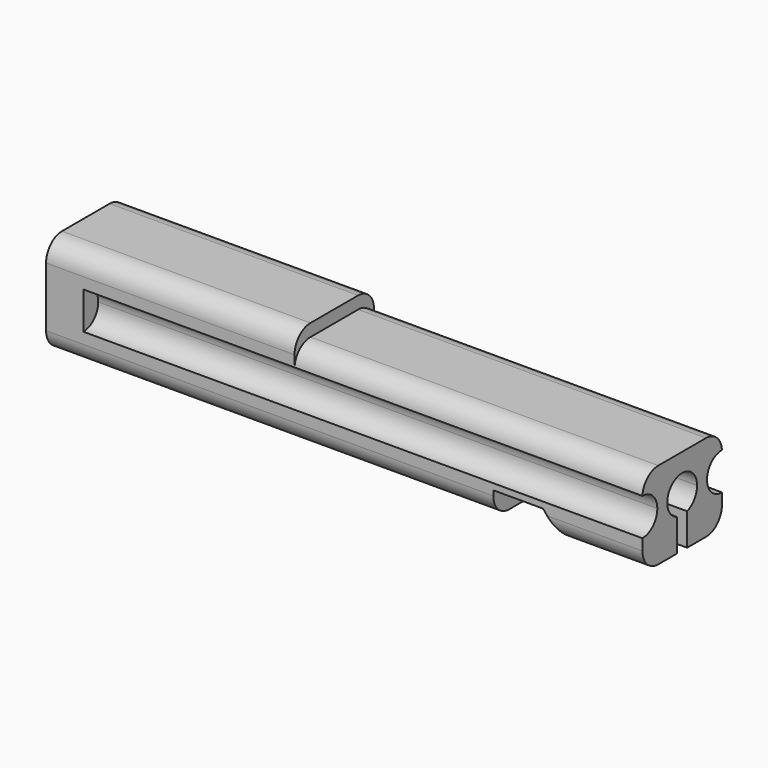
from build123d import *

# Parameters (mm, degrees)
F0_W        = 142.875
F0_H        = 9.525
F1_DEPTH    = 12.7
F3_DEPTH    = 142.875
F5_DEPTH    = 9.525
F6_DEPTH    = 142.875
F7_T1_DEPTH = 101.5751710417
F7_T3_DEPTH = 45.552419836
F7_T5_DEPTH = 139.7
F8_R        = 5.08
F9_DEPTH    = 60.325


# Not quite as in the source:
# - a fillet or chamfer that OpenCascade refuses, or shapes differently, is made with other operations: its cross-section is extruded or revolved along the edge and cut away or added


with BuildPart() as f1:
    # F0 (on Front) → F1 (new body, symmetric)
    with BuildSketch(Plane.XZ):
        Polygon((-20.4177256674, 25.4), (-83.9177256674, 25.4), (-83.9177256674, 0), (30.3822743326, 0), (30.3822743326, 6.35), (43.0822743326, 6.35), (48.3298544966, 0), (68.4822743326, 0), (68.4822743326, 7.9375), (-74.3927256674, 7.9375), (-74.3927256674, 17.4625), (68.4822743326, 17.4625), (68.4822743326, 22.225), (-20.4177256674, 22.225), align=None)
        with Locations((-2.9552256674, 12.7)):
            Rectangle(F0_W, F0_H)
    extrude(amount=F1_DEPTH, both=True)

    # F2 (on face) → F3 (cut)
    with BuildSketch(Plane.YZ.offset(68.4822743326)):
        with BuildLine():
            Line((-4.7625, 12.7), (0, 12.7))
            Line((0, 12.7), (4.7625, 12.7))
            ThreePointArc((4.7625, 12.7), (0, 17.4625), (-4.7625, 12.7))
        make_face()
        with BuildLine():
            Line((-1.5875, 8.2098719395), (0, 8.2098719395))
            Line((0, 8.2098719395), (0, 12.7))
            Line((0, 12.7), (-4.7625, 12.7))
            ThreePointArc((-4.7625, 12.7), (-3.8885649667, 9.950369343), (-1.5875, 8.2098719395))
        make_face()
        with BuildLine():
            ThreePointArc((-1.5875, 8.2098719395), (-0.8053481737, 8.0060868597), (0, 7.9375))
            Line((0, 7.9375), (0, 8.2098719395))
            Line((0, 8.2098719395), (-1.5875, 8.2098719395))
        make_face()
        with BuildLine():
            Line((0, 8.2098719395), (0, 7.9375))
            ThreePointArc((0, 7.9375), (0.8053481737, 8.0060868597), (1.5875, 8.2098719395))
            Line((1.5875, 8.2098719395), (0, 8.2098719395))
        make_face()
        with BuildLine():
            Line((0, 12.7), (0, 8.2098719395))
            Line((0, 8.2098719395), (1.5875, 8.2098719395))
            ThreePointArc((1.5875, 8.2098719395), (3.8885649667, 9.950369343), (4.7625, 12.7))
            Line((4.7625, 12.7), (0, 12.7))
        make_face()
    extrude(amount=-F3_DEPTH, mode=Mode.SUBTRACT)

    # F4 (on face) → F5 (cut)
    with BuildSketch(Plane(origin=(-83.9177256674, 0, 0), x_dir=(0, -1, 0), z_dir=(-1, 0, 0))):
        with BuildLine():
            Line((-0.79375, 12.7), (0.79375, 12.7))
            ThreePointArc((0.79375, 12.7), (0, 13.49375), (-0.79375, 12.7))
        make_face()
        with BuildLine():
            ThreePointArc((-0.79375, 12.7), (0, 11.90625), (0.79375, 12.7))
            Line((0.79375, 12.7), (-0.79375, 12.7))
        make_face()
    extrude(amount=-F5_DEPTH, mode=Mode.SUBTRACT)

    # F2 (on face) → F6 (cut)
    with BuildSketch(Plane.YZ.offset(68.4822743326)):
        with BuildLine():
            ThreePointArc((12.7, 17.4625), (9.3324039546, 16.0675960454), (7.9375, 12.7))
            Line((7.9375, 12.7), (12.7, 12.7))
            Line((12.7, 12.7), (12.7, 17.4625))
        make_face()
        with BuildLine():
            ThreePointArc((7.9375, 12.7), (9.3324039546, 9.3324039546), (12.7, 7.9375))
            Line((12.7, 7.9375), (12.7, 12.7))
            Line((12.7, 12.7), (7.9375, 12.7))
        make_face()
        with BuildLine():
            Line((-12.7, 12.7), (-12.7, 7.9375))
            ThreePointArc((-12.7, 7.9375), (-9.3324039546, 9.3324039546), (-7.9375, 12.7))
            Line((-7.9375, 12.7), (-12.7, 12.7))
        make_face()
        with BuildLine():
            Line((-12.7, 12.7), (-7.9375, 12.7))
            ThreePointArc((-7.9375, 12.7), (-9.3324039546, 16.0675960454), (-12.7, 17.4625))
            Line((-12.7, 17.4625), (-12.7, 12.7))
        make_face()
    extrude(amount=-F6_DEPTH, mode=Mode.SUBTRACT)

    # F7: fillet of radius 5.08 on 6 edges, made by hand

    # F7_s2 → F7_t1 (cut)
    with BuildSketch(Plane.YZ.offset(-20.4177256674)):
        with BuildLine():
            ThreePointArc((7.6299315833, 22.225), (11.1079698235, 20.8476544532), (12.7, 17.4625))
            Line((12.7, 17.4625), (12.7, 22.225))
            Line((12.7, 22.225), (7.6299315833, 22.225))
        make_face()
        with BuildLine():
            ThreePointArc((-7.6299315833, 22.225), (-11.1079698235, 20.8476544532), (-12.7, 17.4625))
            Line((-12.7, 17.4625), (-12.7, 22.225))
            Line((-12.7, 22.225), (-7.6299315833, 22.225))
        make_face()
    extrude(amount=F7_T1_DEPTH, mode=Mode.SUBTRACT)

    # F7_s4 → F7_t3 (cut)
    with BuildSketch(Plane.YZ.offset(35.6298544966)):
        with BuildLine():
            ThreePointArc((12.7, 5.08), (11.2121024484, 1.4878975516), (7.62, 0))
            Line((7.62, 0), (12.7, 0))
            Line((12.7, 0), (12.7, 5.08))
        make_face()
        with BuildLine():
            ThreePointArc((-12.7, 5.08), (-11.2121024484, 1.4878975516), (-7.62, 0))
            Line((-7.62, 0), (-12.7, 0))
            Line((-12.7, 0), (-12.7, 5.08))
        make_face()
    extrude(amount=F7_T3_DEPTH, mode=Mode.SUBTRACT)

    # F7_s6 → F7_t5 (cut)
    with BuildSketch(Plane.YZ.offset(-96.6177256674)):
        with BuildLine():
            ThreePointArc((-12.7, 5.08), (-11.2121024484, 1.4878975516), (-7.62, 0))
            Line((-7.62, 0), (-12.7, 0))
            Line((-12.7, 0), (-12.7, 5.08))
        make_face()
        with BuildLine():
            ThreePointArc((12.7, 5.08), (11.2121024484, 1.4878975516), (7.62, 0))
            Line((7.62, 0), (12.7, 0))
            Line((12.7, 0), (12.7, 5.08))
        make_face()
    extrude(amount=F7_T5_DEPTH, mode=Mode.SUBTRACT)

    # F8
    f8_edges = [f1.edges().sort_by_distance(p)[0] for p in [
        (-52.167726, 12.7, 25.4),
        (-52.167726, -12.7, 25.4),
    ]]
    fillet(f8_edges, radius=F8_R)

    # F2 (on face) → F9 (cut)
    with BuildSketch(Plane.YZ.offset(68.4822743326)):
        with BuildLine():
            Line((0, 7.9375), (0, 0))
            Line((0, 0), (1.5875, 0))
            Line((1.5875, 0), (1.5875, 8.2098719395))
            ThreePointArc((1.5875, 8.2098719395), (0.8053481737, 8.0060868597), (0, 7.9375))
        make_face()
        with BuildLine():
            Line((-1.5875, 0), (0, 0))
            Line((0, 0), (0, 7.9375))
            ThreePointArc((0, 7.9375), (-0.8053481737, 8.0060868597), (-1.5875, 8.2098719395))
            Line((-1.5875, 8.2098719395), (-1.5875, 0))
        make_face()
    extrude(amount=-F9_DEPTH, mode=Mode.SUBTRACT)


solid = f1.part
